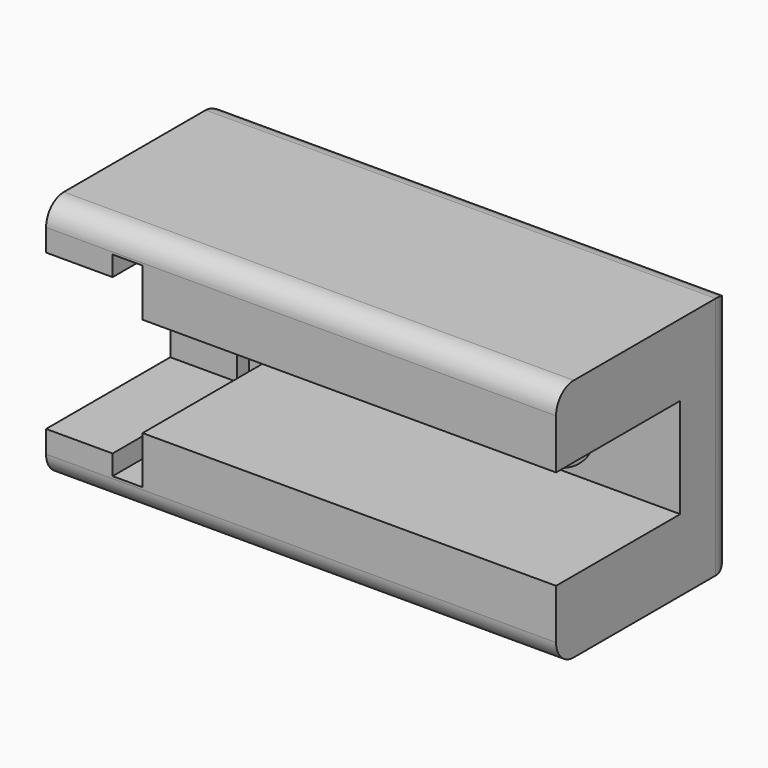
from build123d import *

# Parameters (mm, degrees)
F0_W      = 15
F0_H      = 11
F1_DEPTH  = 10
F2_W      = 15
F2_H      = 4.5
F3_DEPTH  = 7
F4_W      = 3
F4_H      = 7
F5_DEPTH  = 7
F6_W      = 1.35
F6_H      = 8.8
F7_DEPTH  = 7.7
F9_DEPTH  = 8
F10_DEPTH = 8
F11_R     = 1
F12_R     = 1
F13_R     = 2.25
F14_DEPTH = 25


with BuildPart() as f1:
    # F0 (on Front) → F1 (new body)
    with BuildSketch(Plane.XZ):
        Rectangle(F0_W, F0_H)
    extrude(amount=F1_DEPTH)

    # F2 (on face) → F3 (cut)
    with BuildSketch(Plane.XZ.offset(10)):
        Rectangle(F2_W, F2_H)
    extrude(amount=-F3_DEPTH, mode=Mode.SUBTRACT)

    # F4 (on face) → F5 (cut)
    with BuildSketch(Plane.XZ.offset(10)):
        with Locations((-6, 0)):
            Rectangle(F4_W, F4_H)
    extrude(amount=-F5_DEPTH, mode=Mode.SUBTRACT)

    # F6 (on face) → F7 (cut)
    with BuildSketch(Plane.XZ.offset(10)):
        with Locations((-3.825, 0)):
            Rectangle(F6_W, F6_H)
    extrude(amount=-F7_DEPTH, mode=Mode.SUBTRACT)

    # F8 (on face) → F9 (join)
    with BuildSketch(Plane.YZ.offset(7.5)):
        Polygon((-10, 2.25), (-3, 2.25), (0, 2.25), (0, 5.5), (-10, 5.5), align=None)
        Polygon((0, -2.25), (-3, -2.25), (-10, -2.25), (-10, -5.5), (0, -5.5), align=None)
    extrude(amount=F9_DEPTH)

    # F10 (add): a face of the model
    f10_faces = [f1.faces().sort_by_distance(p)[0] for p in [
        (7.5, -1.5, 0),
    ]]
    extrude(f10_faces, amount=F10_DEPTH)

    # F11
    f11_edges = [f1.edges().sort_by_distance(p)[0] for p in [
        (-7.5, 0, 0),
        (4, 0, -5.5),
        (15.5, 0, 0),
        (4, 0, 5.5),
    ]]
    fillet(f11_edges, radius=F11_R)

    # F12
    f12_edges = [f1.edges().sort_by_distance(p)[0] for p in [
        (4, -10, 5.5),
        (4, -1, 5.5),
        (4, -10, -5.5),
        (4, -1, -5.5),
    ]]
    fillet(f12_edges, radius=F12_R)

    # F13 (on face) → F14 (cut)
    with BuildSketch(Plane.XZ.offset(3)):
        with Locations((9.5, 0)):
            Circle(F13_R)
    extrude(amount=-F14_DEPTH, mode=Mode.SUBTRACT)


solid = f1.part
